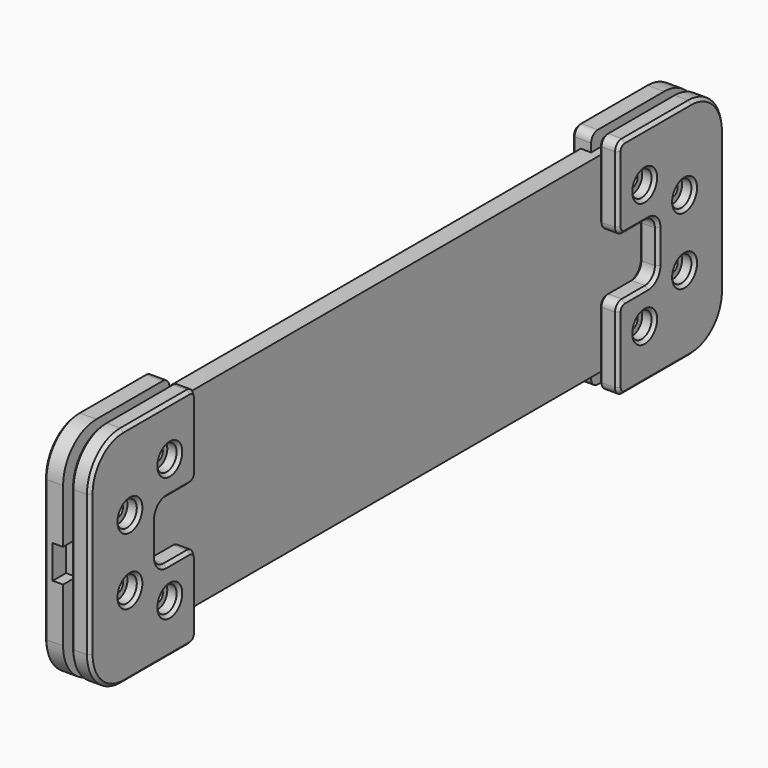
from build123d import *

# Parameters (mm, degrees)
F2_DEPTH  = 2.25
F3_R      = 4.5
F4_DEPTH  = 2.5
F6_DEPTH  = 4.5
F7_R      = 2
F9_DEPTH  = 2
F11_DEPTH = 2.5
F12_R     = 2
F13_R     = 4.25
F14_DEPTH = 4
F15_R     = 1.65
F16_DEPTH = 6.001
F18_DEPTH = 2.4
F19_SIZE  = 0.75
F20_SIZE  = 0.5
F21_R     = 3
F22_DEPTH = 3
F23_R     = 1.65
F24_DEPTH = 8.001
F25_SIZE  = 0.75
F26_SIZE  = 0.5
F27_R     = 1.65
F28_DEPTH = 0.2


# Not quite as in the source:
# - a feature names something its author has since deleted; it is built from what else it names


with BuildPart() as f2:
    # F1 (on Right) → F2 (new body, symmetric)
    with BuildSketch(Plane.YZ):
        with BuildLine():
            Line((85.5, 23), (-85.5, 23))
            ThreePointArc((-85.5, 23), (-89.7426406871, 21.2426406871), (-91.5, 17))
            Line((-91.5, 17), (-91.5, -17))
            ThreePointArc((-91.5, -17), (-89.7426406871, -21.2426406871), (-85.5, -23))
            Line((-85.5, -23), (85.5, -23))
            ThreePointArc((85.5, -23), (89.7426406871, -21.2426406871), (91.5, -17))
            Line((91.5, -17), (91.5, 17))
            ThreePointArc((91.5, 17), (89.7426406871, 21.2426406871), (85.5, 23))
        make_face()
    extrude(amount=F2_DEPTH, both=True)

    # F3 (on Right) → F4 (cut, symmetric)
    with BuildSketch(Plane.YZ):
        with Locations((-83.5, -8)):
            Circle(F3_R)
        with Locations((-71.5, -15)):
            Circle(F3_R)
        with Locations((83.5, -8)):
            Circle(F3_R)
        with Locations((71.5, -15)):
            Circle(F3_R)
        with Locations((83.5, 8)):
            Circle(F3_R)
        with Locations((71.5, 15)):
            Circle(F3_R)
        with Locations((-71.5, 15)):
            Circle(F3_R)
        with Locations((-83.5, 8)):
            Circle(F3_R)
    extrude(amount=F4_DEPTH, both=True, mode=Mode.SUBTRACT)


with BuildPart() as f6:
    # F5 (on face) → F6 (new body)
    with BuildSketch(Plane.YZ.offset(2.25)):
        with BuildLine():
            Line((-75.5, -4), (-75.5, 4))
            ThreePointArc((-75.5, 4), (-74.6213203436, 6.1213203436), (-72.5, 7))
            Line((-72.5, 7), (-63.5, 7))
            Line((-63.5, 7), (-63.5, 27))
            Line((-63.5, 27), (-85.5, 27))
            ThreePointArc((-85.5, 27), (-92.5710678119, 24.0710678119), (-95.5, 17))
            Line((-95.5, 17), (-95.5, -17))
            ThreePointArc((-95.5, -17), (-92.5710678119, -24.0710678119), (-85.5, -27))
            Line((-85.5, -27), (-63.5, -27))
            Line((-63.5, -27), (-63.5, -7))
            Line((-63.5, -7), (-72.5, -7))
            ThreePointArc((-72.5, -7), (-74.6213203436, -6.1213203436), (-75.5, -4))
        make_face()
    extrude(amount=F6_DEPTH)

    # F7
    f7_edges = [f6.edges().sort_by_distance(p)[0] for p in [
        (4.5, -63.5, -7),
        (4.5, -63.5, -27),
        (4.5, -63.5, 7),
        (4.5, -63.5, 27),
    ]]
    fillet(f7_edges, radius=F7_R)

    # F21 (on face) → F22 (cut)
    with BuildSketch(Plane.YZ.offset(6.75)):
        with Locations((-71.5, -15)):
            Circle(F21_R)
        with Locations((-83.5, -8)):
            Circle(F21_R)
        with Locations((-83.5, 8)):
            Circle(F21_R)
        with Locations((-71.5, 15)):
            Circle(F21_R)
    extrude(amount=-F22_DEPTH, mode=Mode.SUBTRACT)

    # F23 (on face) → F24 (cut, through all)
    with BuildSketch(Plane.YZ.offset(3.75)):
        with Locations((-83.5, -8)):
            Circle(F23_R)
        with Locations((-71.5, -15)):
            Circle(F23_R)
        with Locations((-71.5, 15)):
            Circle(F23_R)
        with Locations((-83.5, 8)):
            Circle(F23_R)
    extrude(amount=-F24_DEPTH, mode=Mode.SUBTRACT)

    # F25
    f25_edges = [f6.edges().sort_by_distance(p)[0] for p in [
        (6.75, -75.5, -27),
        (6.75, -64.085786, -26.414214),
        (6.75, -92.571068, -24.071068),
        (6.75, -63.5, -17),
        (6.75, -95.5, 0),
        (6.75, -64.085786, -7.585786),
        (6.75, -92.571068, 24.071068),
        (6.75, -69, -7),
        (6.75, -75.5, 27),
        (6.75, -74.62132, -6.12132),
        (6.75, -64.085786, 26.414214),
        (6.75, -75.5, 0),
        (6.75, -63.5, 17),
        (6.75, -74.62132, 6.12132),
        (6.75, -64.085786, 7.585786),
        (6.75, -69, 7),
        (6.75, -86.5, -8),
        (6.75, -74.5, -15),
        (6.75, -86.5, 8),
        (6.75, -74.5, 15),
    ]]
    chamfer(f25_edges, length=F25_SIZE)

    # F26
    f26_edges = [f6.edges().sort_by_distance(p)[0] for p in [
        (2.25, -75.5, -27),
        (2.25, -64.085786, -26.414214),
        (2.25, -92.571068, -24.071068),
        (2.25, -63.5, -17),
        (2.25, -95.5, 0),
        (2.25, -64.085786, -7.585786),
        (2.25, -92.571068, 24.071068),
        (2.25, -69, -7),
        (2.25, -75.5, 27),
        (2.25, -74.62132, -6.12132),
        (2.25, -64.085786, 26.414214),
        (2.25, -75.5, 0),
        (2.25, -63.5, 17),
        (2.25, -74.62132, 6.12132),
        (2.25, -64.085786, 7.585786),
        (2.25, -69, 7),
        (2.25, -85.15, -8),
        (2.25, -73.15, -15),
        (2.25, -85.15, 8),
        (2.25, -73.15, 15),
    ]]
    chamfer(f26_edges, length=F26_SIZE)


with BuildPart() as f9:
    # F8 (on face) → F9 (new body)
    with BuildSketch(Plane(origin=(-2.25, 0, 0), x_dir=(0, -1, 0), z_dir=(-1, 0, 0))):
        with BuildLine():
            ThreePointArc((75.5, -4), (74.6213203436, -6.1213203436), (72.5, -7))
            Line((72.5, -7), (63.5, -7))
            Line((63.5, -7), (63.5, -27))
            Line((63.5, -27), (85.5, -27))
            ThreePointArc((85.5, -27), (92.5710678119, -24.0710678119), (95.5, -17))
            Line((95.5, -17), (95.5, 0))
            Line((95.5, 0), (95.5, 17))
            ThreePointArc((95.5, 17), (92.5710678119, 24.0710678119), (85.5, 27))
            Line((85.5, 27), (63.5, 27))
            Line((63.5, 27), (63.5, 7))
            Line((63.5, 7), (72.5, 7))
            ThreePointArc((72.5, 7), (74.6213203436, 6.1213203436), (75.5, 4))
            Line((75.5, 4), (75.5, 0))
            Line((75.5, 0), (75.5, -4))
        make_face()
    extrude(amount=F9_DEPTH)

    # F10 (on face) → F11 (join)
    with BuildSketch(Plane.YZ.offset(-2.25)):
        with BuildLine():
            Line((-91.5, -4), (-95.5, -4))
            Line((-95.5, -4), (-95.5, -17))
            ThreePointArc((-95.5, -17), (-92.5710678119, -24.0710678119), (-85.5, -27))
            Line((-85.5, -27), (-63.5, -27))
            Line((-63.5, -27), (-63.5, -23))
            Line((-63.5, -23), (-85.5, -23))
            ThreePointArc((-85.5, -23), (-89.7426406871, -21.2426406871), (-91.5, -17))
            Line((-91.5, -17), (-91.5, -4))
        make_face()
        with BuildLine():
            Line((-63.5, 27), (-85.5, 27))
            ThreePointArc((-85.5, 27), (-92.5710678119, 24.0710678119), (-95.5, 17))
            Line((-95.5, 17), (-95.5, 4))
            Line((-95.5, 4), (-91.5, 4))
            Line((-91.5, 4), (-91.5, 17))
            ThreePointArc((-91.5, 17), (-89.7426406871, 21.2426406871), (-85.5, 23))
            Line((-85.5, 23), (-63.5, 23))
            Line((-63.5, 23), (-63.5, 27))
        make_face()
    extrude(amount=F11_DEPTH)

    # F12
    f12_edges = [f9.edges().sort_by_distance(p)[0] for p in [
        (-2, -63.5, -27),
        (-3.25, -63.5, -7),
        (-3.25, -75.5, -4),
        (-2, -95.5, -17),
        (-2, -63.5, 27),
        (-3.25, -63.5, 7),
    ]]
    fillet(f12_edges, radius=F12_R)

    # F13 (on face) → F14 (join)
    with BuildSketch(Plane.YZ.offset(-2.25)):
        with Locations((-71.5, -15)):
            Circle(F13_R)
        with Locations((-83.5, -8)):
            Circle(F13_R)
        with Locations((-83.5, 8)):
            Circle(F13_R)
        with Locations((-71.5, 15)):
            Circle(F13_R)
    extrude(amount=F14_DEPTH)

    # F15 (on face) → F16 (cut, through all)
    with BuildSketch(Plane.YZ.offset(1.75)):
        with Locations((-71.5, -15)):
            Circle(F15_R)
        with Locations((-83.5, -8)):
            Circle(F15_R)
        with Locations((-71.5, 15)):
            Circle(F15_R)
        with Locations((-83.5, 8)):
            Circle(F15_R)
    extrude(amount=-F16_DEPTH, mode=Mode.SUBTRACT)

    # F17 (on face) → F18 (cut)
    with BuildSketch(Plane(origin=(-4.25, 0, 0), x_dir=(0, -1, 0), z_dir=(-1, 0, 0))):
        Polygon((73.2320508076, -12), (69.7679491924, -12), (68.0358983849, -15), (69.7679491924, -18), (73.2320508076, -18), (74.9641016151, -15), align=None)
        Polygon((83.5, -4.5358983849), (80.5, -6.2679491924), (80.5, -9.7320508076), (83.5, -11.4641016151), (86.5, -9.7320508076), (86.5, -6.2679491924), align=None)
        Polygon((69.7679491924, 18), (68.0358983849, 15), (69.7679491924, 12), (73.2320508076, 12), (74.9641016151, 15), (73.2320508076, 18), align=None)
        Polygon((80.5, 6.2679491924), (83.5, 4.5358983849), (86.5, 6.2679491924), (86.5, 9.7320508076), (83.5, 11.4641016151), (80.5, 9.7320508076), align=None)
    extrude(amount=-F18_DEPTH, mode=Mode.SUBTRACT)

    # F19
    f19_edges = [f9.edges().sort_by_distance(p)[0] for p in [
        (1.75, -75.75, -15),
        (1.75, -87.75, -8),
        (1.75, -87.75, 8),
        (1.75, -75.75, 15),
    ]]
    chamfer(f19_edges, length=F19_SIZE)

    # F20
    f20_edges = [f9.edges().sort_by_distance(p)[0] for p in [
        (-4.25, -69, -7),
        (-4.25, -64.085786, -7.585786),
        (-4.25, -74.62132, -6.12132),
        (-4.25, -63.5, -17),
        (-4.25, -75.5, 0),
        (-4.25, -64.085786, -26.414214),
        (-4.25, -74.62132, 6.12132),
        (-4.25, -75.5, -27),
        (-4.25, -69, 7),
        (-4.25, -92.571068, -24.071068),
        (-4.25, -64.085786, 7.585786),
        (-4.25, -95.5, 0),
        (-4.25, -63.5, 17),
        (-4.25, -92.571068, 24.071068),
        (-4.25, -64.085786, 26.414214),
        (-4.25, -75.5, 27),
        (-4.25, -71.5, -12),
        (-4.25, -68.901924, -13.5),
        (-4.25, -68.901924, -16.5),
        (-4.25, -71.5, -18),
        (-4.25, -74.098076, -16.5),
        (-4.25, -74.098076, -13.5),
        (-4.25, -85, -5.401924),
        (-4.25, -82, -5.401924),
        (-4.25, -80.5, -8),
        (-4.25, -82, -10.598076),
        (-4.25, -85, -10.598076),
        (-4.25, -86.5, -8),
        (-4.25, -68.901924, 16.5),
        (-4.25, -68.901924, 13.5),
        (-4.25, -71.5, 12),
        (-4.25, -74.098076, 13.5),
        (-4.25, -74.098076, 16.5),
        (-4.25, -71.5, 18),
        (-4.25, -80.5, 8),
        (-4.25, -82, 5.401924),
        (-4.25, -85, 5.401924),
        (-4.25, -86.5, 8),
        (-4.25, -85, 10.598076),
        (-4.25, -82, 10.598076),
    ]]
    chamfer(f20_edges, length=F20_SIZE)

    # F27 (on face) → F28 (join)
    with BuildSketch(Plane(origin=(-1.85, 0, 0), x_dir=(0, -1, 0), z_dir=(-1, 0, 0))):
        with Locations((71.5, 15)):
            Circle(F27_R)
        with Locations((83.5, 8)):
            Circle(F27_R)
        with Locations((83.5, -8)):
            Circle(F27_R)
        with Locations((71.5, -15)):
            Circle(F27_R)
    extrude(amount=-F28_DEPTH)


with BuildPart() as f29_1:
    # F29: instance of F6
    add(f6.part.mirror(Plane.XZ))


with BuildPart() as f29_2:
    # F29: instance of F9
    add(f9.part.mirror(Plane.XZ))


solid = Compound([f2.part, f6.part, f9.part, f29_1.part, f29_2.part])
